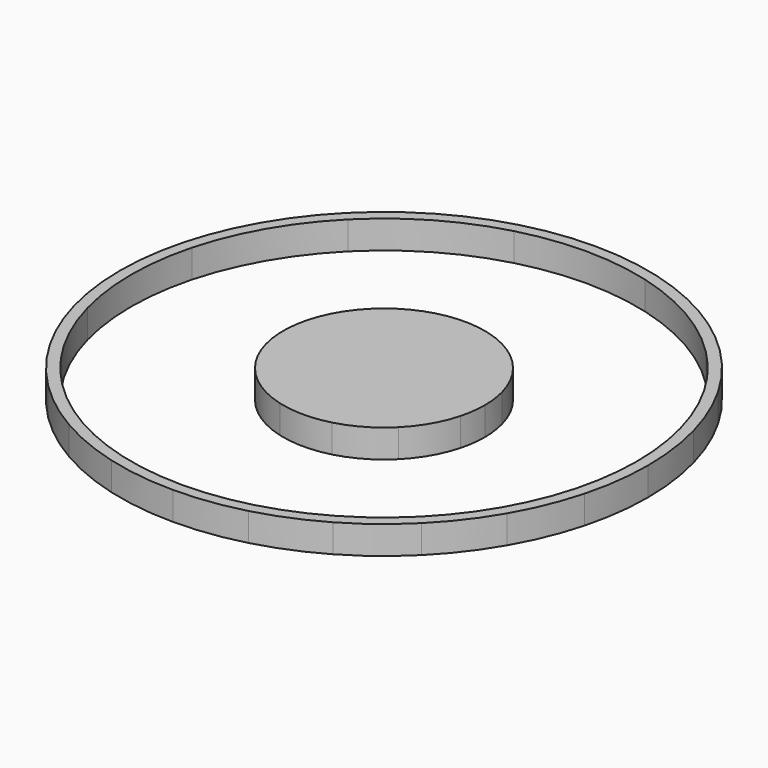
from build123d import *

# Parameters (mm, degrees)
F1_DEPTH = 7


# Not quite as in the source:
# - the program builds the solid bodies; features that only make, move or delete a surface that nothing else refers to are left out


with BuildPart() as f1:
    # F0 (on Top) → F1 (new body)
    with BuildSketch(Plane.XY):
        with BuildLine():
            ThreePointArc((-60.7171979996, 16.2691241707), (-54.4375504652, 31.4295344151), (-44.4480738289, 44.4480738289))
            Line((-44.4480738289, 44.4480738289), (-46.3979145079, 46.3979145079))
            ThreePointArc((-46.3979145079, 46.3979145079), (-52.0571169794, 39.9448308691), (-56.8256077619, 32.8082801112))
            ThreePointArc((-56.8256077619, 32.8082801112), (-60.6217967148, 25.1103704558), (-63.3807299004, 16.9828153925))
            Line((-63.3807299004, 16.9828153925), (-60.7171979996, 16.2691241707))
        make_face()
        with BuildLine():
            ThreePointArc((-44.4480738289, 44.4480738289), (-31.4295344151, 54.4375504652), (-16.2691241707, 60.7171979996))
            Line((-16.2691241707, 60.7171979996), (-16.9828153925, 63.3807299004))
            ThreePointArc((-16.9828153925, 63.3807299004), (-25.110369915, 60.6217969388), (-32.8082790973, 56.8256083472))
            ThreePointArc((-32.8082790973, 56.8256083472), (-39.9448304047, 52.0571173357), (-46.3979145079, 46.3979145079))
            Line((-46.3979145079, 46.3979145079), (-44.4480738289, 44.4480738289))
        make_face()
        with BuildLine():
            ThreePointArc((-16.2691241707, 60.7171979996), (0, 62.8590688303), (16.2691241707, 60.7171979996))
            Line((16.2691241707, 60.7171979996), (16.9828153925, 63.3807299004))
            ThreePointArc((16.9828153925, 63.3807299004), (8.5646797863, 65.0552011873), (1.367e-07, 65.6165599629))
            ThreePointArc((1.367e-07, 65.6165599629), (-8.5646796508, 65.0552012051), (-16.9828153925, 63.3807299004))
            Line((-16.9828153925, 63.3807299004), (-16.2691241707, 60.7171979996))
        make_face()
        with BuildLine():
            Line((44.4480738289, 44.4480738289), (46.3979145079, 46.3979145079))
            ThreePointArc((46.3979145079, 46.3979145079), (39.9448310464, 52.0571168432), (32.8082804984, 56.8256075383))
            ThreePointArc((32.8082804984, 56.8256075383), (25.1103706624, 60.6217966293), (16.9828153925, 63.3807299004))
            Line((16.9828153925, 63.3807299004), (16.2691241707, 60.7171979996))
            ThreePointArc((16.2691241707, 60.7171979996), (31.4295344151, 54.4375504652), (44.4480738289, 44.4480738289))
        make_face()
        with BuildLine():
            Line((-63.3807299004, -16.9828153925), (-60.7171979996, -16.2691241707))
            ThreePointArc((-60.7171979996, -16.2691241707), (-62.8590688303, 0), (-60.7171979996, 16.2691241707))
            Line((-60.7171979996, 16.2691241707), (-63.3807299004, 16.9828153925))
            ThreePointArc((-63.3807299004, 16.9828153925), (-65.0552011962, 8.5646797185), (-65.6165599629, 0))
            ThreePointArc((-65.6165599629, 0), (-65.0552011962, -8.5646797185), (-63.3807299004, -16.9828153925))
        make_face()
        with BuildLine():
            Line((-46.3979145079, -46.3979145079), (-44.4480738289, -44.4480738289))
            ThreePointArc((-44.4480738289, -44.4480738289), (-54.4375504652, -31.4295344151), (-60.7171979996, -16.2691241707))
            Line((-60.7171979996, -16.2691241707), (-63.3807299004, -16.9828153925))
            ThreePointArc((-63.3807299004, -16.9828153925), (-60.6217966456, -25.1103706229), (-56.825607581, -32.8082804245))
            ThreePointArc((-56.825607581, -32.8082804245), (-52.0571168692, -39.9448310126), (-46.3979145079, -46.3979145079))
        make_face()
        with BuildLine():
            Line((-16.9828153925, -63.3807299004), (-16.2691241707, -60.7171979996))
            ThreePointArc((-16.2691241707, -60.7171979996), (-31.4295344151, -54.4375504652), (-44.4480738289, -44.4480738289))
            Line((-44.4480738289, -44.4480738289), (-46.3979145079, -46.3979145079))
            ThreePointArc((-46.3979145079, -46.3979145079), (-39.9448307804, -52.0571170474), (-32.8082799176, -56.8256078737))
            ThreePointArc((-32.8082799176, -56.8256078737), (-25.1103703525, -60.6217967576), (-16.9828153925, -63.3807299004))
        make_face()
        with BuildLine():
            Line((16.9828153925, -63.3807299004), (16.2691241707, -60.7171979996))
            ThreePointArc((16.2691241707, -60.7171979996), (0, -62.8590688303), (-16.2691241707, -60.7171979996))
            Line((-16.2691241707, -60.7171979996), (-16.9828153925, -63.3807299004))
            ThreePointArc((-16.9828153925, -63.3807299004), (-8.5646797185, -65.0552011962), (0, -65.6165599629))
            ThreePointArc((0, -65.6165599629), (8.5646797185, -65.0552011962), (16.9828153925, -63.3807299004))
        make_face()
        with BuildLine():
            ThreePointArc((32.8082803048, -56.8256076501), (39.9448309578, -52.0571169113), (46.3979145079, -46.3979145079))
            Line((46.3979145079, -46.3979145079), (44.4480738289, -44.4480738289))
            ThreePointArc((44.4480738289, -44.4480738289), (31.4295344151, -54.4375504652), (16.2691241707, -60.7171979996))
            Line((16.2691241707, -60.7171979996), (16.9828153925, -63.3807299004))
            ThreePointArc((16.9828153925, -63.3807299004), (25.1103705591, -60.621796672), (32.8082803048, -56.8256076501))
        make_face()
        with BuildLine():
            ThreePointArc((56.8256078737, -32.8082799176), (60.6217967576, -25.1103703525), (63.3807299004, -16.9828153925))
            Line((63.3807299004, -16.9828153925), (60.7171979996, -16.2691241707))
            ThreePointArc((60.7171979996, -16.2691241707), (54.4375504652, -31.4295344151), (44.4480738289, -44.4480738289))
            Line((44.4480738289, -44.4480738289), (46.3979145079, -46.3979145079))
            ThreePointArc((46.3979145079, -46.3979145079), (52.0571170474, -39.9448307804), (56.8256078737, -32.8082799176))
        make_face()
        with BuildLine():
            ThreePointArc((63.3807299004, -16.9828153925), (65.0552011962, -8.5646797185), (65.6165599629, 0))
            ThreePointArc((65.6165599629, 0), (65.0552011962, 8.5646797185), (63.3807299004, 16.9828153925))
            Line((63.3807299004, 16.9828153925), (60.7171979996, 16.2691241707))
            ThreePointArc((60.7171979996, 16.2691241707), (62.3213007825, 8.2047549009), (62.8590688303, 0))
            ThreePointArc((62.8590688303, 0), (62.3213007825, -8.2047549009), (60.7171979996, -16.2691241707))
            Line((60.7171979996, -16.2691241707), (63.3807299004, -16.9828153925))
        make_face()
        with BuildLine():
            Line((60.7171979996, 16.2691241707), (63.3807299004, 16.9828153925))
            ThreePointArc((63.3807299004, 16.9828153925), (60.6217966456, 25.1103706229), (56.825607581, 32.8082804245))
            ThreePointArc((56.825607581, 32.8082804245), (52.0571168692, 39.9448310126), (46.3979145079, 46.3979145079))
            Line((46.3979145079, 46.3979145079), (44.4480738289, 44.4480738289))
            ThreePointArc((44.4480738289, 44.4480738289), (54.4375504652, 31.4295344151), (60.7171979996, 16.2691241707))
        make_face()
    extrude(amount=F1_DEPTH)


with BuildPart() as f1b:
    # F0 (on Top) → F1, piece 2 (new body)
    with BuildSketch(Plane.XY):
        with BuildLine():
            Line((0, 0), (24.1980851045, 6.4838573621))
            ThreePointArc((24.1980851045, 6.4838573621), (21.6954095781, 12.5258505601), (17.7142277423, 17.7142277423))
            Line((17.7142277423, 17.7142277423), (0, 0))
        make_face()
        with BuildLine():
            Line((-6.4838573621, 24.1980851045), (0, 0))
            Line((0, 0), (6.4838573621, 24.1980851045))
            ThreePointArc((6.4838573621, 24.1980851045), (0, 25.0517011202), (-6.4838573621, 24.1980851045))
        make_face()
        with BuildLine():
            Line((-17.7142277423, -17.7142277423), (0, 0))
            Line((0, 0), (-24.1980851045, -6.4838573621))
            ThreePointArc((-24.1980851045, -6.4838573621), (-21.6954095781, -12.5258505601), (-17.7142277423, -17.7142277423))
        make_face()
        with BuildLine():
            Line((-6.4838573621, -24.1980851045), (0, 0))
            Line((0, 0), (-17.7142277423, -17.7142277423))
            ThreePointArc((-17.7142277423, -17.7142277423), (-12.5258505601, -21.6954095781), (-6.4838573621, -24.1980851045))
        make_face()
        with BuildLine():
            Line((6.4838573621, -24.1980851045), (0, 0))
            Line((0, 0), (-6.4838573621, -24.1980851045))
            ThreePointArc((-6.4838573621, -24.1980851045), (0, -25.0517011202), (6.4838573621, -24.1980851045))
        make_face()
        with BuildLine():
            Line((17.7142277423, -17.7142277423), (0, 0))
            Line((0, 0), (6.4838573621, -24.1980851045))
            ThreePointArc((6.4838573621, -24.1980851045), (12.5258505601, -21.6954095781), (17.7142277423, -17.7142277423))
        make_face()
        with BuildLine():
            ThreePointArc((17.7142277423, -17.7142277423), (21.6954095781, -12.5258505601), (24.1980851045, -6.4838573621))
            Line((24.1980851045, -6.4838573621), (0, 0))
            Line((0, 0), (17.7142277423, -17.7142277423))
        make_face()
        with BuildLine():
            ThreePointArc((25.0517011202, 0), (24.8373803443, 3.2699031559), (24.1980851045, 6.4838573621))
            Line((24.1980851045, 6.4838573621), (0, 0))
            Line((0, 0), (24.1980851045, -6.4838573621))
            ThreePointArc((24.1980851045, -6.4838573621), (24.8373803443, -3.2699031559), (25.0517011202, 0))
        make_face()
        with BuildLine():
            Line((-17.7142277423, 17.7142277423), (0, 0))
            Line((0, 0), (-6.4838573621, 24.1980851045))
            ThreePointArc((-6.4838573621, 24.1980851045), (-12.5258505601, 21.6954095781), (-17.7142277423, 17.7142277423))
        make_face()
        with BuildLine():
            Line((-24.1980851045, 6.4838573621), (0, 0))
            Line((0, 0), (-17.7142277423, 17.7142277423))
            ThreePointArc((-17.7142277423, 17.7142277423), (-21.6954095781, 12.5258505601), (-24.1980851045, 6.4838573621))
        make_face()
        with BuildLine():
            Line((-24.1980851045, -6.4838573621), (0, 0))
            Line((0, 0), (-24.1980851045, 6.4838573621))
            ThreePointArc((-24.1980851045, 6.4838573621), (-25.0517011202, 0), (-24.1980851045, -6.4838573621))
        make_face()
        with BuildLine():
            Line((0, 0), (17.7142277423, 17.7142277423))
            ThreePointArc((17.7142277423, 17.7142277423), (12.5258505601, 21.6954095781), (6.4838573621, 24.1980851045))
            Line((6.4838573621, 24.1980851045), (0, 0))
        make_face()
    extrude(amount=F1_DEPTH)


solid = Compound([f1.part, f1b.part])
